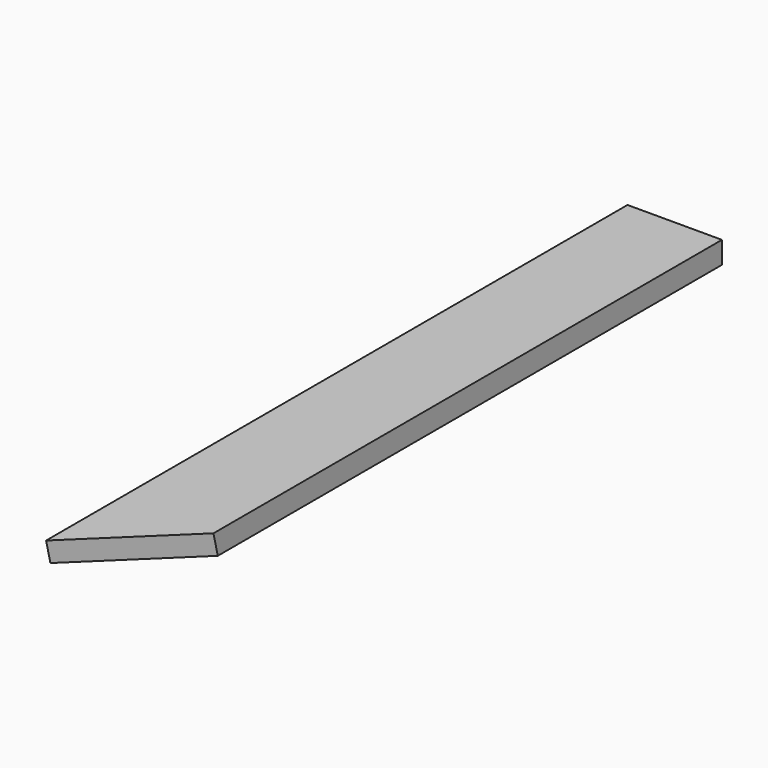
from build123d import *

# Parameters (mm, degrees)
F0_W        = 120
F0_H        = 28
F1_DEPTH    = 462.5
F2_SIZE2    = 115.882643
F2_SIZE     = 119.99999
F3_T1_DEPTH = 343.6641668027


# Not quite as in the source:
# - a fillet or chamfer that OpenCascade refuses, or shapes differently, is made with other operations: its cross-section is extruded or revolved along the edge and cut away or added
# - a fillet or chamfer is up to 0.001 mm smaller than in the source, because OpenCascade refuses the exact size


with BuildPart() as f1:
    # F0 (on Front) → F1 (new body, symmetric)
    with BuildSketch(Plane.XZ):
        Rectangle(F0_W, F0_H)
    extrude(amount=F1_DEPTH, both=True)

    # F2 (size 120 and 115.8826529768 in the source; OpenCascade refuses exactly that, so slightly less here)
    f2_edges = [f1.edges().sort_by_distance(p)[0] for p in [
        (60, -462.5, 0),
    ]]
    f2_side = f1.faces().sort_by_distance((0, -462.5, 0))[0]
    chamfer(f2_edges, length=F2_SIZE, length2=F2_SIZE2, reference=f2_side)

    # F3: chamfer of 6 x 34.0276909177 on 2 edges, made by hand

    # F3_s2 → F3_t1 (cut)
    with BuildSketch(Plane(origin=(-325.7617702656, -314.5844839382, 0), x_dir=(0, 0, 1), z_dir=(0.7193398013, 0.6946583695, 0))):
        Polygon((-14, 285.0151628785), (20.0276909177, 291.0151628785), (-14, 291.0151628785), align=None)
    extrude(amount=F3_T1_DEPTH, mode=Mode.SUBTRACT)


solid = f1.part
